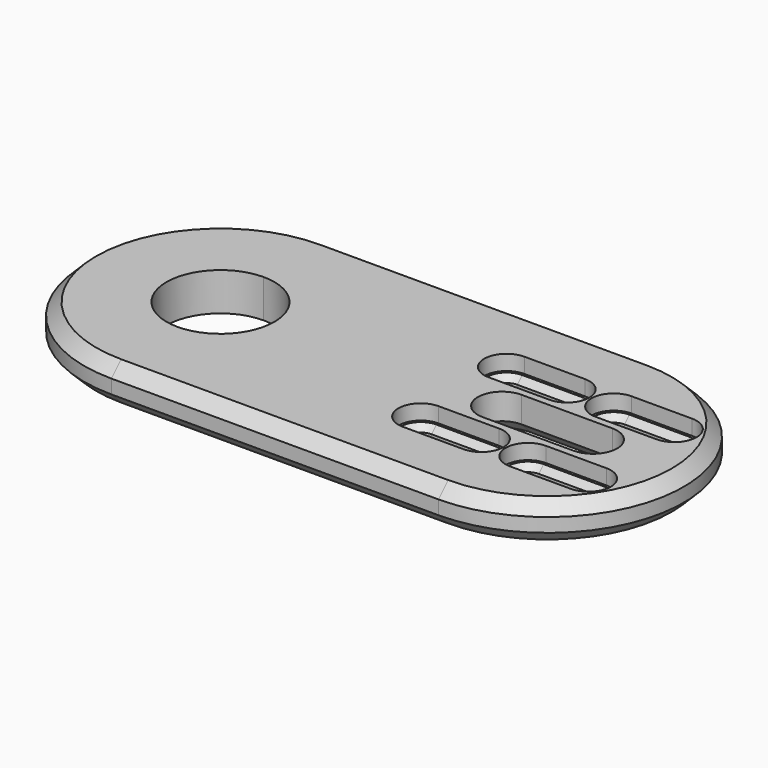
from build123d import *

# Parameters (mm, degrees)
F1_DEPTH = 6.3
F2_SIZE  = 0.5
F3_SIZE  = 2
F4_W     = 10
F4_H     = 0.938
F4_H_2   = 5.5
F5_DEPTH = 2.5
F6_SIZE  = 1
F7_SIZE  = 2


# Not quite as in the source:
# - a feature names something its author has since deleted; it is built from what else it names


with BuildPart() as f1:
    # F0 (on Top) → F1 (new body)
    with BuildSketch(Plane.XY):
        with BuildLine():
            ThreePointArc((27, -22.5), (49.5, 0), (27, 22.5))
            Line((27, 22.5), (27, 4))
            Line((27, 4), (34.5, 4))
            ThreePointArc((34.5, 4), (38.5, 0), (34.5, -4))
            Line((34.5, -4), (27, -4))
            Line((27, -4), (27, -22.5))
        make_face()
        with BuildLine():
            ThreePointArc((30.8505792452, -11.1005792452), (28.6005792452, -8.8505792452), (30.8505792452, -6.6005792452))
            Line((30.8505792452, -6.6005792452), (40.8505792452, -6.6005792452))
            ThreePointArc((40.8505792452, -6.6005792452), (43.1005792452, -8.8505792452), (40.8505792452, -11.1005792452))
            Line((40.8505792452, -11.1005792452), (30.8505792452, -11.1005792452))
        make_face(mode=Mode.SUBTRACT)
        with BuildLine():
            ThreePointArc((30.8505792452, 6.6005792452), (28.6005792452, 8.8505792452), (30.8505792452, 11.1005792452))
            Line((30.8505792452, 11.1005792452), (40.8505792452, 11.1005792452))
            ThreePointArc((40.8505792452, 11.1005792452), (43.1005792452, 8.8505792452), (40.8505792452, 6.6005792452))
            Line((40.8505792452, 6.6005792452), (30.8505792452, 6.6005792452))
        make_face(mode=Mode.SUBTRACT)
        with BuildLine():
            Line((27, 4), (27, 22.5))
            Line((27, 22.5), (-27, 22.5))
            Line((-27, 22.5), (-27, 8.905))
            ThreePointArc((-27, 8.905), (-20.7032141135, 6.2967858865), (-18.095, 0))
            ThreePointArc((-18.095, 0), (-20.7032141135, -6.2967858865), (-27, -8.905))
            Line((-27, -8.905), (-27, -22.5))
            Line((-27, -22.5), (27, -22.5))
            Line((27, -22.5), (27, -4))
            Line((27, -4), (19.5, -4))
            ThreePointArc((19.5, -4), (15.5, 0), (19.5, 4))
            Line((19.5, 4), (27, 4))
        make_face()
        with BuildLine():
            Line((23.1494207548, -11.1005792452), (13.1494207548, -11.1005792452))
            ThreePointArc((13.1494207548, -11.1005792452), (10.8994207548, -8.8505792452), (13.1494207548, -6.6005792452))
            Line((13.1494207548, -6.6005792452), (23.1494207548, -6.6005792452))
            ThreePointArc((23.1494207548, -6.6005792452), (25.3994207548, -8.8505792452), (23.1494207548, -11.1005792452))
        make_face(mode=Mode.SUBTRACT)
        with BuildLine():
            ThreePointArc((13.1494207548, 6.6005792452), (10.8994207548, 8.8505792452), (13.1494207548, 11.1005792452))
            Line((13.1494207548, 11.1005792452), (23.1494207548, 11.1005792452))
            ThreePointArc((23.1494207548, 11.1005792452), (25.3994207548, 8.8505792452), (23.1494207548, 6.6005792452))
            Line((23.1494207548, 6.6005792452), (13.1494207548, 6.6005792452))
        make_face(mode=Mode.SUBTRACT)
        with BuildLine():
            Line((-27, 8.905), (-27, 22.5))
            ThreePointArc((-27, 22.5), (-49.5, 0), (-27, -22.5))
            Line((-27, -22.5), (-27, -8.905))
            ThreePointArc((-27, -8.905), (-35.905, 0), (-27, 8.905))
        make_face()
    extrude(amount=F1_DEPTH)

    # F2
    f2_edges = [f1.edges().sort_by_distance(p)[0] for p in [
        (18.149421, 11.100579, 6.3),
        (35.850579, 11.100579, 6.3),
        (35.850579, -6.600579, 6.3),
        (18.149421, -6.600579, 6.3),
        (35.850579, 11.100579, 0),
        (18.149421, 11.100579, 0),
        (35.850579, -6.600579, 0),
        (18.149421, -6.600579, 0),
        (43.100579, -8.850579, 0),
        (35.850579, -11.100579, 0),
        (28.600579, -8.850579, 0),
        (43.100579, 8.850579, 0),
        (35.850579, 6.600579, 0),
        (28.600579, 8.850579, 0),
        (18.149421, 6.600579, 0),
        (10.899421, 8.850579, 0),
        (25.399421, 8.850579, 0),
        (18.149421, -11.100579, 0),
        (10.899421, -8.850579, 0),
        (25.399421, -8.850579, 0),
    ]]
    chamfer(f2_edges, length=F2_SIZE)

    # F3
    f3_edges = [f1.edges().sort_by_distance(p)[0] for p in [
        (0, -22.5, 6.3),
        (0, -22.5, 0),
    ]]
    chamfer(f3_edges, length=F3_SIZE)

    # F4 (on face) → F5 (cut)
    with BuildSketch(Plane.XY.offset(6.3)):
        with Locations((18.1494207548, 12.0695792452)):
            Rectangle(F4_W, F4_H)
        with BuildLine():
            Line((13.1494207548, 11.6005792452), (13.1494207548, 12.5385792452))
            ThreePointArc((13.1494207548, 12.5385792452), (9.4614207548, 8.8505792452), (13.1494207548, 5.1625792452))
            Line((13.1494207548, 5.1625792452), (13.1494207548, 6.1005792452))
            ThreePointArc((13.1494207548, 6.1005792452), (10.3994207548, 8.8505792452), (13.1494207548, 11.6005792452))
        make_face()
        with BuildLine():
            Line((13.1494207548, 6.1005792452), (13.1494207548, 11.6005792452))
            ThreePointArc((13.1494207548, 11.6005792452), (10.3994207548, 8.8505792452), (13.1494207548, 6.1005792452))
        make_face()
        with Locations((18.1494207548, 8.8505792452)):
            Rectangle(F4_W, F4_H_2)
        with Locations((18.1494207548, 5.6315792452)):
            Rectangle(F4_W, F4_H)
        with BuildLine():
            ThreePointArc((23.1494207548, 6.1005792452), (25.8994207548, 8.8505792452), (23.1494207548, 11.6005792452))
            Line((23.1494207548, 11.6005792452), (23.1494207548, 6.1005792452))
        make_face()
        with BuildLine():
            ThreePointArc((23.1494207548, 5.1625792452), (26.8374207548, 8.8505792452), (23.1494207548, 12.5385792452))
            Line((23.1494207548, 12.5385792452), (23.1494207548, 11.6005792452))
            ThreePointArc((23.1494207548, 11.6005792452), (25.8994207548, 8.8505792452), (23.1494207548, 6.1005792452))
            Line((23.1494207548, 6.1005792452), (23.1494207548, 5.1625792452))
        make_face()
        with BuildLine():
            ThreePointArc((30.8505792452, 12.5385792452), (27.1625792452, 8.8505792452), (30.8505792452, 5.1625792452))
            Line((30.8505792452, 5.1625792452), (30.8505792452, 6.1005792452))
            ThreePointArc((30.8505792452, 6.1005792452), (28.1005792452, 8.8505792452), (30.8505792452, 11.6005792452))
            Line((30.8505792452, 11.6005792452), (30.8505792452, 12.5385792452))
        make_face()
        with BuildLine():
            ThreePointArc((30.8505792452, 11.6005792452), (28.1005792452, 8.8505792452), (30.8505792452, 6.1005792452))
            Line((30.8505792452, 6.1005792452), (30.8505792452, 11.6005792452))
        make_face()
        with Locations((35.8505792452, 8.8505792452)):
            Rectangle(F4_W, F4_H_2)
        with Locations((35.8505792452, 12.0695792452)):
            Rectangle(F4_W, F4_H)
        with Locations((35.8505792452, 5.6315792452)):
            Rectangle(F4_W, F4_H)
        with BuildLine():
            Line((40.8505792452, 6.1005792452), (40.8505792452, 5.1625792452))
            ThreePointArc((40.8505792452, 5.1625792452), (44.5385792452, 8.8505792452), (40.8505792452, 12.5385792452))
            Line((40.8505792452, 12.5385792452), (40.8505792452, 11.6005792452))
            ThreePointArc((40.8505792452, 11.6005792452), (43.6005792452, 8.8505792452), (40.8505792452, 6.1005792452))
        make_face()
        with BuildLine():
            Line((40.8505792452, 11.6005792452), (40.8505792452, 6.1005792452))
            ThreePointArc((40.8505792452, 6.1005792452), (43.6005792452, 8.8505792452), (40.8505792452, 11.6005792452))
        make_face()
        with Locations((18.1494207548, -8.8505792452)):
            Rectangle(F4_W, F4_H_2)
        with BuildLine():
            ThreePointArc((13.1494207548, -6.1005792452), (10.3994207548, -8.8505792452), (13.1494207548, -11.6005792452))
            Line((13.1494207548, -11.6005792452), (13.1494207548, -6.1005792452))
        make_face()
        with BuildLine():
            Line((23.1494207548, -6.1005792452), (23.1494207548, -11.6005792452))
            ThreePointArc((23.1494207548, -11.6005792452), (25.8994207548, -8.8505792452), (23.1494207548, -6.1005792452))
        make_face()
        with Locations((18.1494207548, -5.6315792452)):
            Rectangle(F4_W, F4_H)
        with BuildLine():
            Line((23.1494207548, -11.6005792452), (23.1494207548, -12.5385792452))
            ThreePointArc((23.1494207548, -12.5385792452), (26.8374207548, -8.8505792452), (23.1494207548, -5.1625792452))
            Line((23.1494207548, -5.1625792452), (23.1494207548, -6.1005792452))
            ThreePointArc((23.1494207548, -6.1005792452), (25.8994207548, -8.8505792452), (23.1494207548, -11.6005792452))
        make_face()
        with Locations((18.1494207548, -12.0695792452)):
            Rectangle(F4_W, F4_H)
        with BuildLine():
            ThreePointArc((13.1494207548, -5.1625792452), (9.4614207548, -8.8505792452), (13.1494207548, -12.5385792452))
            Line((13.1494207548, -12.5385792452), (13.1494207548, -11.6005792452))
            ThreePointArc((13.1494207548, -11.6005792452), (10.3994207548, -8.8505792452), (13.1494207548, -6.1005792452))
            Line((13.1494207548, -6.1005792452), (13.1494207548, -5.1625792452))
        make_face()
        with BuildLine():
            ThreePointArc((30.8505792452, -5.1625792452), (27.1625792452, -8.8505792452), (30.8505792452, -12.5385792452))
            Line((30.8505792452, -12.5385792452), (30.8505792452, -11.6005792452))
            ThreePointArc((30.8505792452, -11.6005792452), (28.1005792452, -8.8505792452), (30.8505792452, -6.1005792452))
            Line((30.8505792452, -6.1005792452), (30.8505792452, -5.1625792452))
        make_face()
        with Locations((35.8505792452, -5.6315792452)):
            Rectangle(F4_W, F4_H)
        with Locations((35.8505792452, -8.8505792452)):
            Rectangle(F4_W, F4_H_2)
        with Locations((35.8505792452, -12.0695792452)):
            Rectangle(F4_W, F4_H)
        with BuildLine():
            ThreePointArc((30.8505792452, -6.1005792452), (28.1005792452, -8.8505792452), (30.8505792452, -11.6005792452))
            Line((30.8505792452, -11.6005792452), (30.8505792452, -6.1005792452))
        make_face()
        with BuildLine():
            Line((40.8505792452, -6.1005792452), (40.8505792452, -11.6005792452))
            ThreePointArc((40.8505792452, -11.6005792452), (43.6005792452, -8.8505792452), (40.8505792452, -6.1005792452))
        make_face()
        with BuildLine():
            Line((40.8505792452, -11.6005792452), (40.8505792452, -12.5385792452))
            ThreePointArc((40.8505792452, -12.5385792452), (44.5385792452, -8.8505792452), (40.8505792452, -5.1625792452))
            Line((40.8505792452, -5.1625792452), (40.8505792452, -6.1005792452))
            ThreePointArc((40.8505792452, -6.1005792452), (43.6005792452, -8.8505792452), (40.8505792452, -11.6005792452))
        make_face()
    extrude(amount=-F5_DEPTH, mode=Mode.SUBTRACT)

    # F6
    f6_edges = [f1.edges().sort_by_distance(p)[0] for p in [
        (10.899421, 8.850579, 3.8),
        (18.149421, 6.600579, 3.8),
        (25.399421, 8.850579, 3.8),
        (18.149421, 11.100579, 3.8),
        (35.850579, 11.100579, 3.8),
        (28.600579, 8.850579, 3.8),
        (43.100579, 8.850579, 3.8),
        (35.850579, 6.600579, 3.8),
        (35.850579, -6.600579, 3.8),
        (28.600579, -8.850579, 3.8),
        (43.100579, -8.850579, 3.8),
        (35.850579, -11.100579, 3.8),
        (18.149421, -6.600579, 3.8),
        (10.899421, -8.850579, 3.8),
        (25.399421, -8.850579, 3.8),
        (18.149421, -11.100579, 3.8),
    ]]
    chamfer(f6_edges, length=F6_SIZE)

    # F7
    f7_edges = [f1.edges().sort_by_distance(p)[0] for p in [
        (27, 4, 0),
        (38.5, 0, 0),
        (27, -4, 0),
        (15.5, 0, 0),
    ]]
    chamfer(f7_edges, length=F7_SIZE)


solid = f1.part
